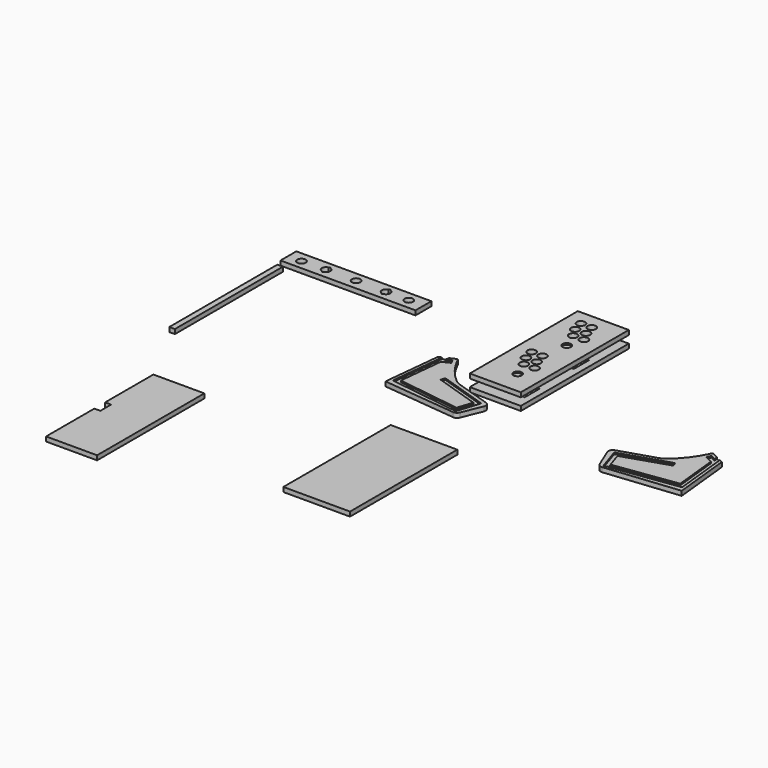
from build123d import *

# Parameters (mm, degrees)
F0_W     = 450
F0_H     = 66
F0_R     = 14
F1_DEPTH = 15
F0_W_2   = 222.18
F0_H_2   = 446.9934681001
F0_W_3   = 18.6
F0_H_3   = 450
F0_W_4   = 170
F2_DEPTH = 10
F3_DEPTH = 3
F4_START = 40
F4_DEPTH = 15
F5_START = 40
F5_DEPTH = 10


# Not quite as in the source:
# - ends of sketch curves that miss each other by under 0.0002 mm in the source are joined
# - a feature names something its author has since deleted; it is built from what else it names


with BuildPart() as f1:
    # F0 (on Top) → F1 (new body)
    with BuildSketch(Plane.XY):
        with Locations((-275.3125, 174.566393)):
            Rectangle(F0_W, F0_H)
        with Locations((-455.3125, 172.667105)):
            Circle(F0_R, mode=Mode.SUBTRACT)
        with BuildLine():
            ThreePointArc((-378.2477990597, 189.0446940126), (-375.3124995108, 191.425001), (-372.3772007381, 189.0446930553))
            ThreePointArc((-372.3772007381, 189.0446930553), (-361.3125360954, 175.3889517933), (-372.3125330795, 161.6810653625))
            ThreePointArc((-372.3125330795, 161.6810653625), (-375.3124999977, 158.667106), (-378.3124675242, 161.6810649978))
            ThreePointArc((-378.3124675242, 161.6810649978), (-389.3124649032, 175.3889523889), (-378.2477990597, 189.0446940126))
        make_face(mode=Mode.SUBTRACT)
        with Locations((-275.3125, 175.355867)):
            Circle(F0_R, mode=Mode.SUBTRACT)
        with BuildLine():
            ThreePointArc((-178.2477990597, 189.0446940126), (-175.3124995108, 191.425001), (-172.3772007381, 189.0446930553))
            ThreePointArc((-172.3772007381, 189.0446930553), (-161.3125360966, 175.3889522817), (-172.3125321254, 161.6810655718))
            ThreePointArc((-172.3125321254, 161.6810655718), (-175.3125000023, 158.667106), (-178.3124675242, 161.6810650024))
            ThreePointArc((-178.3124675242, 161.6810650024), (-189.3124649043, 175.3889519005), (-178.2477990597, 189.0446940126))
        make_face(mode=Mode.SUBTRACT)
        with Locations((-99.3125, 175.046053)):
            Circle(F0_R, mode=Mode.SUBTRACT)
    extrude(amount=F1_DEPTH)


with BuildPart() as f1b:
    # F0 (on Top) → F1, piece 2 (new body)
    with BuildSketch(Plane.XY):
        with Locations((414.0754595661, -627.1019588439)):
            Rectangle(F0_W_2, F0_H_2)
    extrude(amount=F1_DEPTH)


with BuildPart() as f1c:
    # F0 (on Top) → F1, piece 3 (new body)
    with BuildSketch(Plane.XY):
        with Locations((-482.7783352852, -107.0080339909)):
            Rectangle(F0_W_3, F0_H_3)
    extrude(amount=F1_DEPTH)


with BuildPart() as f1d:
    # F0 (on Top) → F1, piece 4 (new body)
    with BuildSketch(Plane.XY):
        Polygon((-357.1018981934, -813.1195902824), (-357.1018981934, -1014.1163243325), (-187.1018981934, -1014.1163243325), (-187.1018981934, -567.1228562324), (-357.1018981934, -567.1228562324), (-357.1018981934, -768.1195902824), (-337.1018981934, -768.1195902824), (-337.1018981934, -813.1195902824), align=None)
    extrude(amount=F1_DEPTH)


with BuildPart() as f1e:
    # F0 (on Top) → F1, piece 5 (new body)
    with BuildSketch(Plane.XY):
        with Locations((415.3125, 117.075)):
            Rectangle(F0_W_4, F0_H_3)
        Polygon((398.896491766, -63.403442502), (379.896491766, -63.403442502), (379.896491766, -42.903442502), (379.896491766, -20.903442502), (379.896491766, -0.403442502), (398.896491766, -0.403442502), (458.896491766, -0.403442502), (477.896491766, -0.403442502), (477.896491766, -20.903442502), (477.896491766, -42.903442502), (477.896491766, -63.403442502), (458.896491766, -63.403442502), align=None, mode=Mode.SUBTRACT)
        with Locations((407.3125, 21.075)):
            Circle(F0_R, mode=Mode.SUBTRACT)
        with Locations((389.3125, 52.325)):
            Circle(F0_R, mode=Mode.SUBTRACT)
        with Locations((380.3125, 87.325)):
            Circle(F0_R, mode=Mode.SUBTRACT)
        with Locations((443.3125, 21.075)):
            Circle(F0_R, mode=Mode.SUBTRACT)
        with Locations((425.3125, 52.325)):
            Circle(F0_R, mode=Mode.SUBTRACT)
        with Locations((416.3125, 87.325)):
            Circle(F0_R, mode=Mode.SUBTRACT)
        Polygon((379.896491766, 183.4961353032), (379.896491766, 203.9961353032), (398.896491766, 203.9961353032), (458.896491766, 203.9961353032), (477.896491766, 203.9961353032), (477.896491766, 183.4961353032), (477.896491766, 161.4961353032), (477.896491766, 140.9961353032), (458.896491766, 140.9961353032), (398.896491766, 140.9961353032), (379.896491766, 140.9961353032), (379.896491766, 161.4961353032), align=None, mode=Mode.SUBTRACT)
        with Locations((407.3125, 226.325)):
            Circle(F0_R, mode=Mode.SUBTRACT)
        with Locations((443.3125, 226.325)):
            Circle(F0_R, mode=Mode.SUBTRACT)
        with Locations((389.3125, 257.575)):
            Circle(F0_R, mode=Mode.SUBTRACT)
        with Locations((380.3125, 292.575)):
            Circle(F0_R, mode=Mode.SUBTRACT)
        with Locations((425.3125, 257.575)):
            Circle(F0_R, mode=Mode.SUBTRACT)
        with Locations((416.3125, 292.575)):
            Circle(F0_R, mode=Mode.SUBTRACT)
    extrude(amount=F1_DEPTH)

    # F0 (on Top) → F2 (join)
    with BuildSketch(Plane.XY):
        Polygon((379.896491766, -0.403442502), (379.896491766, -20.903442502), (389.396491766, -20.903442502), (398.896491766, -10.653442502), (398.896491766, -0.403442502), align=None)
        Polygon((468.396491766, -20.903442502), (477.896491766, -20.903442502), (477.896491766, -0.403442502), (458.896491766, -0.403442502), (458.896491766, -10.653442502), align=None)
        Polygon((379.896491766, -42.903442502), (379.896491766, -63.403442502), (398.896491766, -63.403442502), (398.896491766, -53.153442502), (389.396491766, -42.903442502), align=None)
        Polygon((458.896491766, -53.153442502), (458.896491766, -63.403442502), (477.896491766, -63.403442502), (477.896491766, -42.903442502), (468.396491766, -42.903442502), align=None)
        Polygon((398.896491766, 203.9961353032), (379.896491766, 203.9961353032), (379.896491766, 183.4961353032), (389.396491766, 183.4961353032), (398.896491766, 193.7461353032), align=None)
        Polygon((477.896491766, 203.9961353032), (458.896491766, 203.9961353032), (458.896491766, 193.7461353032), (468.396491766, 183.4961353032), (477.896491766, 183.4961353032), align=None)
        Polygon((389.396491766, 161.4961353032), (379.896491766, 161.4961353032), (379.896491766, 140.9961353032), (398.896491766, 140.9961353032), (398.896491766, 151.2461353032), align=None)
        Polygon((477.896491766, 140.9961353032), (477.896491766, 161.4961353032), (468.396491766, 161.4961353032), (458.896491766, 151.2461353032), (458.896491766, 140.9961353032), align=None)
    extrude(amount=F2_DEPTH)

    # F3 (add): faces of the model
    f3_faces = [f1e.faces().sort_by_distance(p)[0] for p in [
        (388.4917298612, 194.7223257794, 10),
        (388.4917298612, 150.2699448271, 10),
        (469.3012536707, 194.7223257794, 10),
        (469.3012536707, 150.2699448271, 10),
        (388.4917298612, -9.6772520258, 10),
        (388.4917298612, -54.1296329782, 10),
        (469.3012536707, -54.1296329782, 10),
        (469.3012536707, -9.6772520258, 10),
    ]]
    extrude(f3_faces, amount=-F3_DEPTH)


with BuildPart() as f1f:
    # F0 (on Top) → F1, piece 6 (new body)
    with BuildSketch(Plane.XY):
        with BuildLine():
            ThreePointArc((302.5028120746, -113.4118397649), (291.7895222642, -108.8231641307), (282.1654510284, -102.249901966))
            ThreePointArc((282.1654510284, -102.249901966), (242.4270473876, -61.0976923381), (212.2735658759, -12.4827523493))
            Line((212.2735658759, -12.4827523493), (212.3753570131, -12.4331054945))
            Line((212.3753570131, -12.4331054945), (210.1835012807, -7.9391352623))
            ThreePointArc((210.1835012807, -7.9391352623), (207.3173718223, -5.4033981173), (203.497675316, -5.6370207625))
            Line((203.497675316, -5.6370207625), (185.3208903686, -14.5024311294))
            Line((185.3208903686, -14.5024311294), (184.1050070735, -26.2214764388))
            Line((184.1050070735, -26.2214764388), (201.0889002444, -17.9378782655))
            Line((201.0889002444, -17.9378782655), (207.6644674419, -31.4197889621))
            Line((207.6644674419, -31.4197889621), (182.2811821308, -43.8000444029))
            Line((182.2811821308, -43.8000444029), (167.0090810672, -190.9971027505))
            Line((167.0090810672, -190.9971027505), (372.719644, -219.907837))
            Line((372.719644, -219.907837), (370.632048, -234.761858))
            Line((370.632048, -234.761858), (165.4600818342, -205.9268186771))
            Line((165.4600818342, -205.9268186771), (150.5962994139, -203.8378502933))
            Line((150.5962994139, -203.8378502933), (169.4365677719, -22.2497329007))
            Line((169.4365677719, -22.2497329007), (158.8470193741, -27.4146007482))
            Line((158.8470193741, -27.4146007482), (138.8807909164, -219.8550569122))
            Line((138.8807909164, -219.8550569122), (384.285849, -245.316509))
            ThreePointArc((384.285849, -245.316509), (393.5291994484, -243.272206896), (399.7074436243, -236.0994808456))
            Line((399.7074436243, -236.0994808456), (426.902704, -169.940574))
            ThreePointArc((426.902704, -169.940574), (426.6214042378, -157.893477256), (417.5678269321, -149.9408422138))
            Line((417.5678269321, -149.9408422138), (302.5028120746, -113.4118397649))
        make_face()
        Polygon((406.3898916745, -175.2648505781), (386.03579, -237.908333), (371.769942, -233.273078), (392.124043671, -170.6295955888), (244.880684, -122.787328), (249.515939, -108.521481), (411.195547, -161.05437), (406.560292, -175.320217), align=None, mode=Mode.SUBTRACT)
    extrude(amount=F1_DEPTH)

    # F0 (on Top) → F2, piece 2 (join)
    with BuildSketch(Plane.XY):
        Polygon((406.430912, -175.138603), (406.3898916745, -175.2648505781), (406.560292, -175.320217), (411.195547, -161.05437), (249.515939, -108.521481), (244.880684, -122.787328), (392.124043671, -170.6295955888), (392.165064, -170.503348), align=None)
        Polygon((371.769942, -233.273078), (386.03579, -237.908333), (406.3898916745, -175.2648505781), (392.124043671, -170.6295955888), align=None)
        Polygon((184.1050070735, -26.2214764388), (185.3208903686, -14.5024311294), (169.4365677719, -22.2497329007), (150.5962994139, -203.8378502933), (165.4600818342, -205.9268186771), (167.0090810672, -190.9971027505), (182.2811821308, -43.8000444029), align=None)
        Polygon((201.0889002444, -17.9378782655), (184.1050070735, -26.2214764388), (182.2811821308, -43.8000444029), (207.6644674419, -31.4197889621), align=None)
        Polygon((167.0090810672, -190.9971027505), (165.4600818342, -205.9268186771), (370.632048, -234.761858), (372.719644, -219.907837), align=None)
        Polygon((392.124043671, -170.6295955888), (406.3898916745, -175.2648505781), (406.430912, -175.138603), (392.165064, -170.503348), align=None)
    extrude(amount=F2_DEPTH)


with BuildPart() as f1g:
    # F0 (on Top) → F1, piece 7 (new body)
    with BuildSketch(Plane.XY):
        with BuildLine():
            Line((1054.9340247737, -7.9391352623), (1052.7421690412, -12.4331054945))
            Line((1052.7421690412, -12.4331054945), (1052.8439601784, -12.4827523493))
            ThreePointArc((1052.8439601784, -12.4827523493), (1022.6904786668, -61.0976923381), (982.9520768924, -102.2499008063))
            ThreePointArc((982.9520768924, -102.2499008063), (973.3280037901, -108.8231641307), (962.6147139797, -113.4118397649))
            Line((962.6147139797, -113.4118397649), (847.5496990544, -149.940842))
            ThreePointArc((847.5496990544, -149.940842), (838.4961218165, -157.893477256), (838.2148214301, -169.9405738456))
            Line((838.2148214301, -169.9405738456), (865.4100830544, -236.099481))
            ThreePointArc((865.4100830544, -236.099481), (871.588326606, -243.272206896), (880.8316770801, -245.316509248))
            Line((880.8316770801, -245.316509248), (1126.236735138, -219.8550569122))
            Line((1126.236735138, -219.8550569122), (1106.2705066803, -27.4146007482))
            Line((1106.2705066803, -27.4146007482), (1095.6809582825, -22.2497329007))
            Line((1095.6809582825, -22.2497329007), (1114.5212266405, -203.8378502933))
            Line((1114.5212266405, -203.8378502933), (1099.6574442202, -205.9268186771))
            Line((1099.6574442202, -205.9268186771), (894.4854780544, -234.761858))
            Line((894.4854780544, -234.761858), (892.3978820544, -219.907837))
            Line((892.3978820544, -219.907837), (1098.1084449872, -190.9971027505))
            Line((1098.1084449872, -190.9971027505), (1082.8363439236, -43.8000444029))
            Line((1082.8363439236, -43.8000444029), (1057.4530586125, -31.4197889621))
            Line((1057.4530586125, -31.4197889621), (1064.02862581, -17.9378782655))
            Line((1064.02862581, -17.9378782655), (1081.0125189809, -26.2214764388))
            Line((1081.0125189809, -26.2214764388), (1079.7966356858, -14.5024311294))
            Line((1079.7966356858, -14.5024311294), (1061.6198507384, -5.6370207625))
            ThreePointArc((1061.6198507384, -5.6370207625), (1057.8001542321, -5.4033981173), (1054.9340247737, -7.9391352623))
        make_face()
        Polygon((1020.2368420544, -122.787328), (872.9934823834, -170.6295955888), (893.3475840544, -233.273078), (879.0817360544, -237.908333), (858.7276343799, -175.2648505781), (858.5572340544, -175.320217), (853.9219790544, -161.05437), (1015.6015870544, -108.521481), align=None, mode=Mode.SUBTRACT)
    extrude(amount=F1_DEPTH)

    # F0 (on Top) → F2, piece 3 (join)
    with BuildSketch(Plane.XY):
        Polygon((1095.6809582825, -22.2497329007), (1079.7966356858, -14.5024311294), (1081.0125189809, -26.2214764388), (1082.8363439236, -43.8000444029), (1098.1084449872, -190.9971027505), (1099.6574442202, -205.9268186771), (1114.5212266405, -203.8378502933), align=None)
        Polygon((894.4854780544, -234.761858), (1099.6574442202, -205.9268186771), (1098.1084449872, -190.9971027505), (892.3978820544, -219.907837), align=None)
        Polygon((893.3475840544, -233.273078), (872.9934823834, -170.6295955888), (858.7276343799, -175.2648505781), (879.0817360544, -237.908333), align=None)
        Polygon((858.6866140544, -175.138603), (872.9524620544, -170.503348), (872.9934823834, -170.6295955888), (1020.2368420544, -122.787328), (1015.6015870544, -108.521481), (853.9219790544, -161.05437), (858.5572340544, -175.320217), (858.7276343799, -175.2648505781), align=None)
        Polygon((872.9934823834, -170.6295955888), (872.9524620544, -170.503348), (858.6866140544, -175.138603), (858.7276343799, -175.2648505781), align=None)
        Polygon((1082.8363439236, -43.8000444029), (1081.0125189809, -26.2214764388), (1064.02862581, -17.9378782655), (1057.4530586125, -31.4197889621), align=None)
    extrude(amount=F2_DEPTH)


with BuildPart() as f4:
    # F0 (on Top) → F4 (new body)
    with BuildSketch(Plane.XY.offset(F4_START)):
        with Locations((415.3125, 117.075)):
            Rectangle(F0_W_4, F0_H_3)
        Polygon((398.896491766, -63.403442502), (379.896491766, -63.403442502), (379.896491766, -42.903442502), (379.896491766, -20.903442502), (379.896491766, -0.403442502), (398.896491766, -0.403442502), (458.896491766, -0.403442502), (477.896491766, -0.403442502), (477.896491766, -20.903442502), (477.896491766, -42.903442502), (477.896491766, -63.403442502), (458.896491766, -63.403442502), align=None, mode=Mode.SUBTRACT)
        with Locations((407.3125, 21.075)):
            Circle(F0_R, mode=Mode.SUBTRACT)
        with Locations((389.3125, 52.325)):
            Circle(F0_R, mode=Mode.SUBTRACT)
        with Locations((380.3125, 87.325)):
            Circle(F0_R, mode=Mode.SUBTRACT)
        with Locations((443.3125, 21.075)):
            Circle(F0_R, mode=Mode.SUBTRACT)
        with Locations((425.3125, 52.325)):
            Circle(F0_R, mode=Mode.SUBTRACT)
        with Locations((416.3125, 87.325)):
            Circle(F0_R, mode=Mode.SUBTRACT)
        Polygon((379.896491766, 183.4961353032), (379.896491766, 203.9961353032), (398.896491766, 203.9961353032), (458.896491766, 203.9961353032), (477.896491766, 203.9961353032), (477.896491766, 183.4961353032), (477.896491766, 161.4961353032), (477.896491766, 140.9961353032), (458.896491766, 140.9961353032), (398.896491766, 140.9961353032), (379.896491766, 140.9961353032), (379.896491766, 161.4961353032), align=None, mode=Mode.SUBTRACT)
        with Locations((407.3125, 226.325)):
            Circle(F0_R, mode=Mode.SUBTRACT)
        with Locations((443.3125, 226.325)):
            Circle(F0_R, mode=Mode.SUBTRACT)
        with Locations((389.3125, 257.575)):
            Circle(F0_R, mode=Mode.SUBTRACT)
        with Locations((380.3125, 292.575)):
            Circle(F0_R, mode=Mode.SUBTRACT)
        with Locations((425.3125, 257.575)):
            Circle(F0_R, mode=Mode.SUBTRACT)
        with Locations((416.3125, 292.575)):
            Circle(F0_R, mode=Mode.SUBTRACT)
        Polygon((458.896491766, 203.9961353032), (398.896491766, 203.9961353032), (398.896491766, 193.7461353032), (389.396491766, 183.4961353032), (379.896491766, 183.4961353032), (379.896491766, 161.4961353032), (389.396491766, 161.4961353032), (398.896491766, 151.2461353032), (398.896491766, 140.9961353032), (458.896491766, 140.9961353032), (458.896491766, 151.2461353032), (468.396491766, 161.4961353032), (477.896491766, 161.4961353032), (477.896491766, 183.4961353032), (468.396491766, 183.4961353032), (458.896491766, 193.7461353032), align=None)
        with Locations((428.896491766, 172.4961353032)):
            Circle(F0_R, mode=Mode.SUBTRACT)
        Polygon((398.896491766, -53.153442502), (398.896491766, -63.403442502), (458.896491766, -63.403442502), (458.896491766, -53.153442502), (468.396491766, -42.903442502), (477.896491766, -42.903442502), (477.896491766, -20.903442502), (468.396491766, -20.903442502), (458.896491766, -10.653442502), (458.896491766, -0.403442502), (398.896491766, -0.403442502), (398.896491766, -10.653442502), (389.396491766, -20.903442502), (379.896491766, -20.903442502), (379.896491766, -42.903442502), (389.396491766, -42.903442502), align=None)
        with Locations((428.896491766, -31.903442502)):
            Circle(F0_R, mode=Mode.SUBTRACT)
        Polygon((389.396491766, 161.4961353032), (379.896491766, 161.4961353032), (379.896491766, 140.9961353032), (398.896491766, 140.9961353032), (398.896491766, 151.2461353032), align=None)
        Polygon((477.896491766, 203.9961353032), (458.896491766, 203.9961353032), (458.896491766, 193.7461353032), (468.396491766, 183.4961353032), (477.896491766, 183.4961353032), align=None)
        Polygon((398.896491766, 203.9961353032), (379.896491766, 203.9961353032), (379.896491766, 183.4961353032), (389.396491766, 183.4961353032), (398.896491766, 193.7461353032), align=None)
        Polygon((477.896491766, 140.9961353032), (477.896491766, 161.4961353032), (468.396491766, 161.4961353032), (458.896491766, 151.2461353032), (458.896491766, 140.9961353032), align=None)
        Polygon((468.396491766, -20.903442502), (477.896491766, -20.903442502), (477.896491766, -0.403442502), (458.896491766, -0.403442502), (458.896491766, -10.653442502), align=None)
        Polygon((458.896491766, -53.153442502), (458.896491766, -63.403442502), (477.896491766, -63.403442502), (477.896491766, -42.903442502), (468.396491766, -42.903442502), align=None)
        Polygon((379.896491766, -0.403442502), (379.896491766, -20.903442502), (389.396491766, -20.903442502), (398.896491766, -10.653442502), (398.896491766, -0.403442502), align=None)
        Polygon((379.896491766, -42.903442502), (379.896491766, -63.403442502), (398.896491766, -63.403442502), (398.896491766, -53.153442502), (389.396491766, -42.903442502), align=None)
    extrude(amount=F4_DEPTH)

    # F0 (on Top) → F5 (cut)
    with BuildSketch(Plane.XY.offset(F5_START)):
        Polygon((379.896491766, -0.403442502), (379.896491766, -20.903442502), (389.396491766, -20.903442502), (398.896491766, -10.653442502), (398.896491766, -0.403442502), align=None)
        Polygon((398.896491766, -53.153442502), (398.896491766, -63.403442502), (458.896491766, -63.403442502), (458.896491766, -53.153442502), (468.396491766, -42.903442502), (477.896491766, -42.903442502), (477.896491766, -20.903442502), (468.396491766, -20.903442502), (458.896491766, -10.653442502), (458.896491766, -0.403442502), (398.896491766, -0.403442502), (398.896491766, -10.653442502), (389.396491766, -20.903442502), (379.896491766, -20.903442502), (379.896491766, -42.903442502), (389.396491766, -42.903442502), align=None)
        with Locations((428.896491766, -31.903442502)):
            Circle(F0_R, mode=Mode.SUBTRACT)
        Polygon((379.896491766, -42.903442502), (379.896491766, -63.403442502), (398.896491766, -63.403442502), (398.896491766, -53.153442502), (389.396491766, -42.903442502), align=None)
        Polygon((458.896491766, -53.153442502), (458.896491766, -63.403442502), (477.896491766, -63.403442502), (477.896491766, -42.903442502), (468.396491766, -42.903442502), align=None)
        Polygon((468.396491766, -20.903442502), (477.896491766, -20.903442502), (477.896491766, -0.403442502), (458.896491766, -0.403442502), (458.896491766, -10.653442502), align=None)
        Polygon((398.896491766, 203.9961353032), (379.896491766, 203.9961353032), (379.896491766, 183.4961353032), (389.396491766, 183.4961353032), (398.896491766, 193.7461353032), align=None)
        Polygon((389.396491766, 161.4961353032), (379.896491766, 161.4961353032), (379.896491766, 140.9961353032), (398.896491766, 140.9961353032), (398.896491766, 151.2461353032), align=None)
        Polygon((458.896491766, 203.9961353032), (398.896491766, 203.9961353032), (398.896491766, 193.7461353032), (389.396491766, 183.4961353032), (379.896491766, 183.4961353032), (379.896491766, 161.4961353032), (389.396491766, 161.4961353032), (398.896491766, 151.2461353032), (398.896491766, 140.9961353032), (458.896491766, 140.9961353032), (458.896491766, 151.2461353032), (468.396491766, 161.4961353032), (477.896491766, 161.4961353032), (477.896491766, 183.4961353032), (468.396491766, 183.4961353032), (458.896491766, 193.7461353032), align=None)
        with Locations((428.896491766, 172.4961353032)):
            Circle(F0_R, mode=Mode.SUBTRACT)
        Polygon((477.896491766, 140.9961353032), (477.896491766, 161.4961353032), (468.396491766, 161.4961353032), (458.896491766, 151.2461353032), (458.896491766, 140.9961353032), align=None)
        Polygon((477.896491766, 203.9961353032), (458.896491766, 203.9961353032), (458.896491766, 193.7461353032), (468.396491766, 183.4961353032), (477.896491766, 183.4961353032), align=None)
    extrude(amount=F5_DEPTH, mode=Mode.SUBTRACT)


solid = Compound([f1.part, f1b.part, f1c.part, f1d.part, f1e.part, f1f.part, f1g.part, f4.part])
